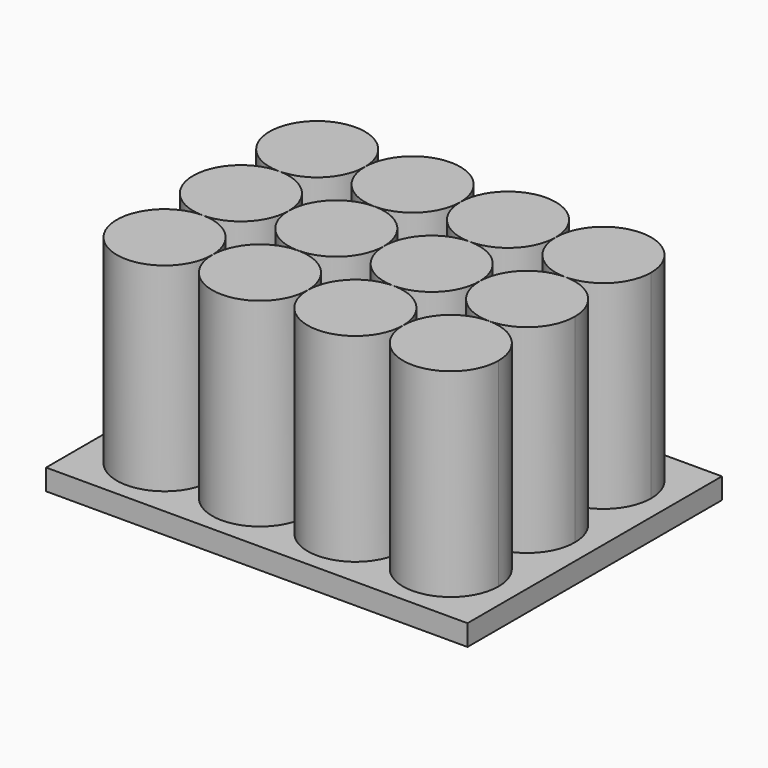
from build123d import *

# Parameters (mm, degrees)
F1_DEPTH = 63.5
F2_W     = 134.62
F2_H     = 6.6927933697
F3_DEPTH = 50.8


# Not quite as in the source:
# - a feature names something its author has since deleted; it is built from what else it names


with BuildPart() as f1:
    # F0 (on Top) → F1 (new body)
    with BuildSketch(Plane.XY):
        with BuildLine():
            ThreePointArc((-45.72, -15.24), (-56.4963073453, -41.2563073453), (-30.48, -30.48))
            ThreePointArc((-30.48, -30.48), (-34.9436926547, -19.7036926547), (-45.72, -15.24))
        make_face()
    extrude(amount=F1_DEPTH)


with BuildPart() as f1b:
    # F0 (on Top) → F1, piece 2 (new body)
    with BuildSketch(Plane.XY):
        with BuildLine():
            ThreePointArc((-15.2399999801, -15.24), (-26.0163073382, -19.7036926477), (-30.48, -30.48))
            ThreePointArc((-30.48, -30.48), (-15.24, -45.72), (0, -30.48))
            ThreePointArc((0, -30.48), (-4.4636926477, -19.7036926618), (-15.2399999801, -15.24))
        make_face()
    extrude(amount=F1_DEPTH)


with BuildPart() as f1c:
    # F0 (on Top) → F1, piece 3 (new body)
    with BuildSketch(Plane.XY):
        with BuildLine():
            ThreePointArc((-45.72, 15.24), (-60.96, 0), (-45.72, -15.24))
            ThreePointArc((-45.72, -15.24), (-34.9436926547, -10.7763073453), (-30.48, 0))
            ThreePointArc((-30.48, 0), (-34.9436926547, 10.7763073453), (-45.72, 15.24))
        make_face()
    extrude(amount=F1_DEPTH)


with BuildPart() as f1d:
    # F0 (on Top) → F1, piece 4 (new body)
    with BuildSketch(Plane.XY):
        with BuildLine():
            ThreePointArc((15.2400000199, -15.24), (4.4636926618, -19.7036926477), (0, -30.48))
            ThreePointArc((0, -30.48), (15.24, -45.72), (30.48, -30.48))
            ThreePointArc((30.48, -30.48), (26.0163073523, -19.7036926618), (15.2400000199, -15.24))
        make_face()
    extrude(amount=F1_DEPTH)


with BuildPart() as f1e:
    # F0 (on Top) → F1, piece 5 (new body)
    with BuildSketch(Plane.XY):
        with BuildLine():
            ThreePointArc((-30.48, 0), (-26.0163073382, -10.7763073523), (-15.2399999801, -15.24))
            ThreePointArc((-15.2399999801, -15.24), (-4.4636926477, -10.7763073382), (0, 0))
            ThreePointArc((0, 0), (-4.4636926477, 10.7763073382), (-15.2399999801, 15.24))
            ThreePointArc((-15.2399999801, 15.24), (-26.0163073382, 10.7763073523), (-30.48, 0))
        make_face()
    extrude(amount=F1_DEPTH)


with BuildPart() as f1f:
    # F0 (on Top) → F1, piece 6 (new body)
    with BuildSketch(Plane.XY):
        with BuildLine():
            ThreePointArc((-30.48, 30.48), (-56.4963073453, 41.2563073453), (-45.72, 15.24))
            ThreePointArc((-45.72, 15.24), (-34.9436926547, 19.7036926547), (-30.48, 30.48))
        make_face()
    extrude(amount=F1_DEPTH)


with BuildPart() as f1g:
    # F0 (on Top) → F1, piece 7 (new body)
    with BuildSketch(Plane.XY):
        with BuildLine():
            ThreePointArc((45.7200000919, -15.24), (34.9436926872, -19.7036926222), (30.48, -30.48))
            ThreePointArc((30.48, -30.48), (45.72, -45.72), (60.96, -30.48))
            ThreePointArc((60.96, -30.48), (56.4963073778, -19.7036926872), (45.7200000919, -15.24))
        make_face()
    extrude(amount=F1_DEPTH)


with BuildPart() as f1h:
    # F0 (on Top) → F1, piece 8 (new body)
    with BuildSketch(Plane.XY):
        with BuildLine():
            ThreePointArc((0, 0), (4.4636926618, -10.7763073523), (15.2400000199, -15.24))
            ThreePointArc((15.2400000199, -15.24), (26.0163073523, -10.7763073382), (30.48, 0))
            ThreePointArc((30.48, 0), (26.0163073523, 10.7763073382), (15.2400000199, 15.24))
            ThreePointArc((15.2400000199, 15.24), (4.4636926618, 10.7763073523), (0, 0))
        make_face()
    extrude(amount=F1_DEPTH)


with BuildPart() as f1i:
    # F0 (on Top) → F1, piece 9 (new body)
    with BuildSketch(Plane.XY):
        with BuildLine():
            ThreePointArc((0, 30.48), (-15.24, 45.72), (-30.48, 30.48))
            ThreePointArc((-30.48, 30.48), (-26.0163073382, 19.7036926477), (-15.2399999801, 15.24))
            ThreePointArc((-15.2399999801, 15.24), (-4.4636926477, 19.7036926618), (0, 30.48))
        make_face()
    extrude(amount=F1_DEPTH)


with BuildPart() as f1j:
    # F0 (on Top) → F1, piece 10 (new body)
    with BuildSketch(Plane.XY):
        with BuildLine():
            ThreePointArc((30.48, 0), (34.9436926872, -10.7763073778), (45.7200000919, -15.24))
            ThreePointArc((45.7200000919, -15.24), (56.4963073778, -10.7763073128), (60.96, 0))
            ThreePointArc((60.96, 0), (56.4963073778, 10.7763073128), (45.7200000919, 15.24))
            ThreePointArc((45.7200000919, 15.24), (34.9436926872, 10.7763073778), (30.48, 0))
        make_face()
    extrude(amount=F1_DEPTH)


with BuildPart() as f1k:
    # F0 (on Top) → F1, piece 11 (new body)
    with BuildSketch(Plane.XY):
        with BuildLine():
            ThreePointArc((0, 30.48), (4.4636926618, 19.7036926477), (15.2400000199, 15.24))
            ThreePointArc((15.2400000199, 15.24), (26.0163073523, 19.7036926618), (30.48, 30.48))
            ThreePointArc((30.48, 30.48), (15.24, 45.72), (0, 30.48))
        make_face()
    extrude(amount=F1_DEPTH)


with BuildPart() as f1l:
    # F0 (on Top) → F1, piece 12 (new body)
    with BuildSketch(Plane.XY):
        with BuildLine():
            ThreePointArc((30.48, 30.48), (34.9436926872, 19.7036926222), (45.7200000919, 15.24))
            ThreePointArc((45.7200000919, 15.24), (56.4963073778, 19.7036926872), (60.96, 30.48))
            ThreePointArc((60.96, 30.48), (45.72, 45.72), (30.48, 30.48))
        make_face()
    extrude(amount=F1_DEPTH)


with BuildPart() as f3:
    # F2 (on Front) → F3 (new body, symmetric)
    with BuildSketch(Plane.XZ):
        with Locations((0, -3.3463966849)):
            Rectangle(F2_W, F2_H)
    extrude(amount=F3_DEPTH, both=True)


solid = Compound([f1.part, f1b.part, f1c.part, f1d.part, f1e.part, f1f.part, f1g.part, f1h.part, f1i.part, f1j.part, f1k.part, f1l.part, f3.part])
